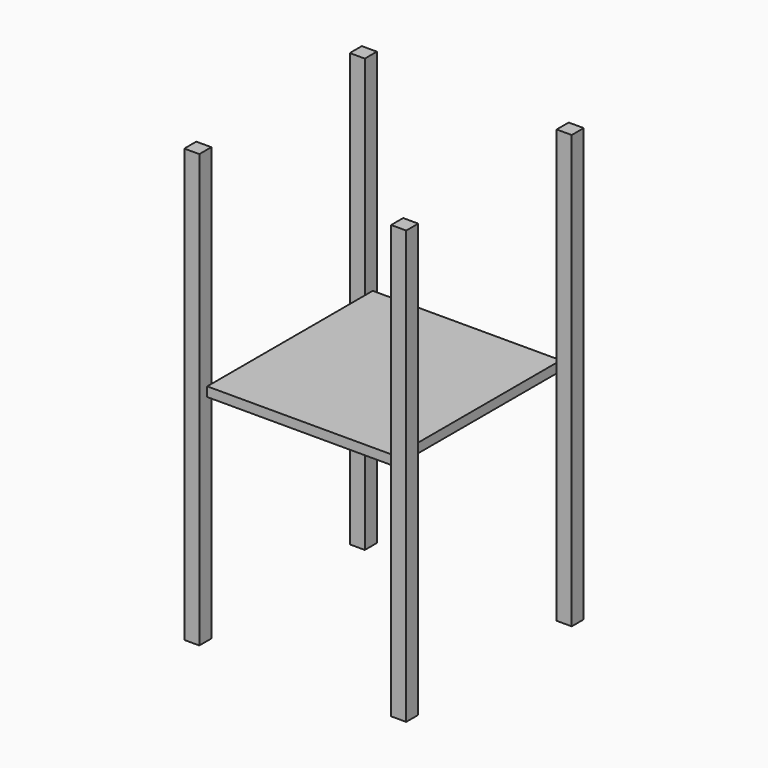
from build123d import *

# Parameters (mm, degrees)
F0_W     = 8
F0_H     = 8
F1_DEPTH = 230
F3_W     = 100
F3_H     = 110
F4_DEPTH = 5


# Not quite as in the source:
# - the program builds the solid bodies; features that only make, move or delete a surface that nothing else refers to are left out


with BuildPart() as f1:
    # F0 (on Top) → F1 (new body)
    with BuildSketch(Plane.XY):
        with Locations((-55, 55)):
            Rectangle(F0_W, F0_H)
    extrude(amount=F1_DEPTH)


with BuildPart() as f1b:
    # F0 (on Top) → F1, piece 2 (new body)
    with BuildSketch(Plane.XY):
        with Locations((-55, -55)):
            Rectangle(F0_W, F0_H)
    extrude(amount=F1_DEPTH)


with BuildPart() as f1c:
    # F0 (on Top) → F1, piece 3 (new body)
    with BuildSketch(Plane.XY):
        with Locations((55, 55)):
            Rectangle(F0_W, F0_H)
    extrude(amount=F1_DEPTH)


with BuildPart() as f1d:
    # F0 (on Top) → F1, piece 4 (new body)
    with BuildSketch(Plane.XY):
        with Locations((55, -55)):
            Rectangle(F0_W, F0_H)
    extrude(amount=F1_DEPTH)


with BuildPart() as f4:
    # F3 (on offset) → F4 (new body)
    with BuildSketch(Plane.XY.offset(120)):
        Rectangle(F3_W, F3_H)
    extrude(amount=-F4_DEPTH)


solid = Compound([f1.part, f1b.part, f1c.part, f1d.part, f4.part])
